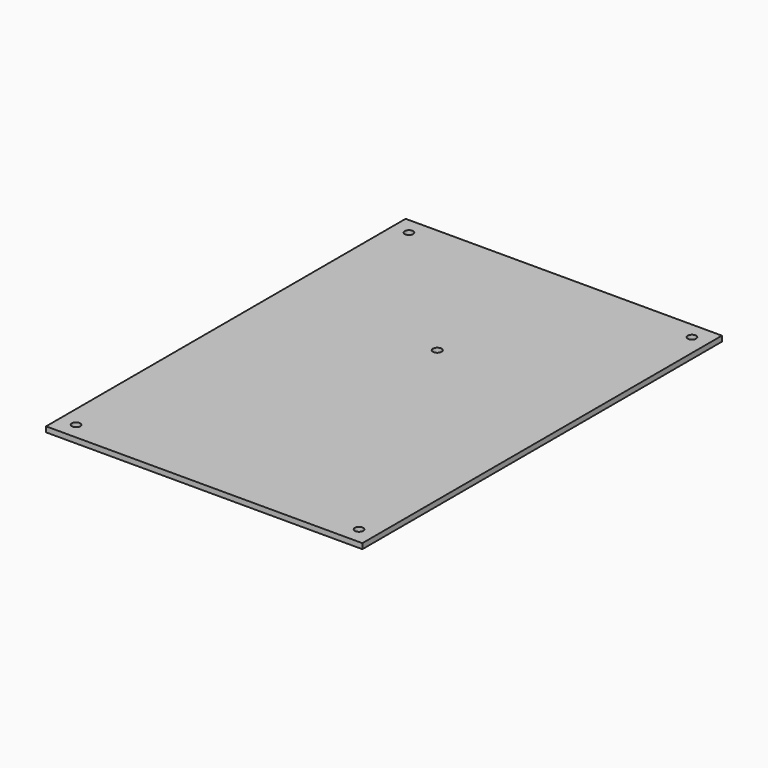
from build123d import *

# Parameters (mm, degrees)
F0_W     = 190
F0_H     = 270
F0_R     = 2.5
F0_R_2   = 80
F0_R_3   = 2.6
F1_DEPTH = 3.2


# Not quite as in the source:
# - a feature names something its author has since deleted; it is built from what else it names


with BuildPart() as f1:
    # F0 (on Top) → F1 (new body)
    with BuildSketch(Plane.XY):
        Rectangle(F0_W, F0_H)
        with Locations((-85, -125)):
            Circle(F0_R, mode=Mode.SUBTRACT)
        with Locations((85, -125)):
            Circle(F0_R, mode=Mode.SUBTRACT)
        with Locations((-85, 125)):
            Circle(F0_R, mode=Mode.SUBTRACT)
        with Locations((0, 40)):
            Circle(F0_R_2, mode=Mode.SUBTRACT)
        with Locations((85, 125)):
            Circle(F0_R, mode=Mode.SUBTRACT)
        with Locations((0, 40)):
            Circle(F0_R_2)
        with Locations((0, 40)):
            Circle(F0_R_3, mode=Mode.SUBTRACT)
    extrude(amount=F1_DEPTH)


solid = f1.part
